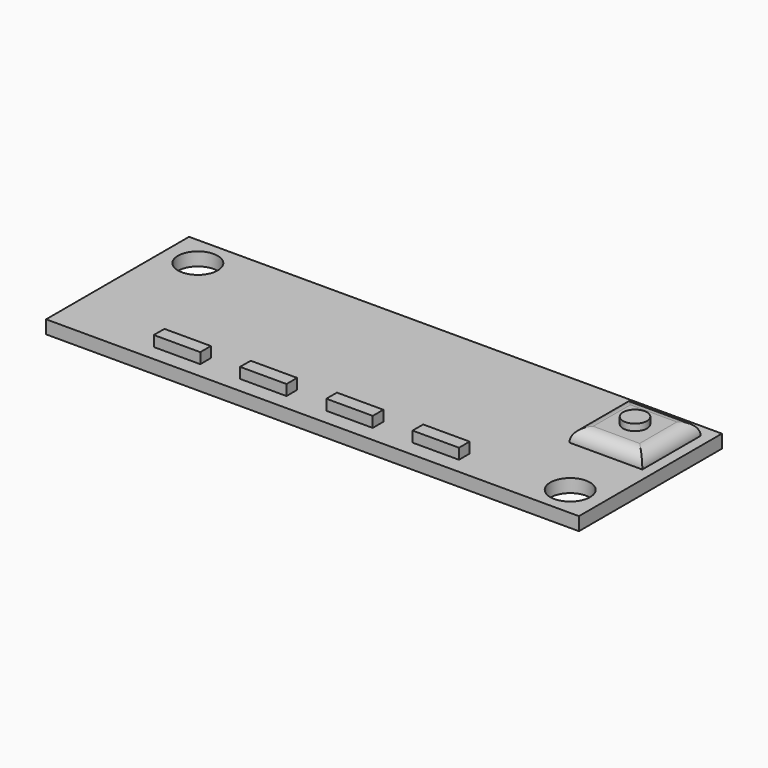
from build123d import *

# Parameters (mm, degrees)
F0_W     = 40.16
F0_H     = 13.47
F0_W_2   = 3.5
F0_H_2   = 1
F0_R     = 1.5
F0_W_3   = 5.5
F0_H_3   = 5.5
F1_DEPTH = 1
F2_DEPTH = 1.8
F3_DEPTH = 2
F4_R     = 0.99999
F5_R     = 0.9
F6_DEPTH = 0.5
F7_W     = 3
F7_H     = 8.5
F8_DEPTH = 1.2


# Not quite as in the source:
# - a fillet or chamfer is up to 0.001 mm smaller than in the source, because OpenCascade refuses the exact size


with BuildPart() as f1:
    # F0 (on Top) → F1 (new body)
    with BuildSketch(Plane.XY):
        with Locations((1.9053274065, 3.3154582972)):
            Rectangle(F0_W, F0_H)
        with Locations((-9.2646725935, -1.7195417028)):
            Rectangle(F0_W_2, F0_H_2, mode=Mode.SUBTRACT)
        with Locations((-2.7646725935, -1.7195417028)):
            Rectangle(F0_W_2, F0_H_2, mode=Mode.SUBTRACT)
        with Locations((3.7353274065, -1.7195417028)):
            Rectangle(F0_W_2, F0_H_2, mode=Mode.SUBTRACT)
        with Locations((10.2353274065, -1.7195417028)):
            Rectangle(F0_W_2, F0_H_2, mode=Mode.SUBTRACT)
        with Locations((19.4853274065, -1.1195417028)):
            Circle(F0_R, mode=Mode.SUBTRACT)
        with Locations((-15.6746725935, 7.7504582972)):
            Circle(F0_R, mode=Mode.SUBTRACT)
        with Locations((18.4353274065, 6.3004582972)):
            Rectangle(F0_W_3, F0_H_3, mode=Mode.SUBTRACT)
        with Locations((-9.2646725935, -1.7195417028)):
            Rectangle(F0_W_2, F0_H_2)
        with Locations((-2.7646725935, -1.7195417028)):
            Rectangle(F0_W_2, F0_H_2)
        with Locations((3.7353274065, -1.7195417028)):
            Rectangle(F0_W_2, F0_H_2)
        with Locations((10.2353274065, -1.7195417028)):
            Rectangle(F0_W_2, F0_H_2)
        with Locations((18.4353274065, 6.3004582972)):
            Rectangle(F0_W_3, F0_H_3)
    extrude(amount=F1_DEPTH)

    # F0 (on Top) → F2 (join)
    with BuildSketch(Plane.XY):
        with Locations((-9.2646725935, -1.7195417028)):
            Rectangle(F0_W_2, F0_H_2)
        with Locations((-2.7646725935, -1.7195417028)):
            Rectangle(F0_W_2, F0_H_2)
        with Locations((3.7353274065, -1.7195417028)):
            Rectangle(F0_W_2, F0_H_2)
        with Locations((10.2353274065, -1.7195417028)):
            Rectangle(F0_W_2, F0_H_2)
    extrude(amount=F2_DEPTH)

    # F0 (on Top) → F3 (join)
    with BuildSketch(Plane.XY):
        with Locations((18.4353274065, 6.3004582972)):
            Rectangle(F0_W_3, F0_H_3)
    extrude(amount=F3_DEPTH)

    # F4 (radius 1 in the source; OpenCascade refuses exactly that, so slightly less here)
    f4_edges = [f1.edges().sort_by_distance(p)[0] for p in [
        (21.185327, 6.300458, 2),
        (15.685327, 6.300458, 2),
        (18.435327, 3.550458, 2),
        (18.435327, 9.050458, 2),
    ]]
    fillet(f4_edges, radius=F4_R)

    # F5 (on face) → F6 (join)
    with BuildSketch(Plane.XY.offset(2)):
        with Locations((18.4353274065, 6.3004582972)):
            Circle(F5_R)
    extrude(amount=F6_DEPTH)

    # F7 (on face) → F8 (join)
    with BuildSketch(Plane(origin=(0, 0, 0), x_dir=(1, 0, 0), z_dir=(0, 0, -1))):
        with Locations((-1.5146725935, -4.8004582972)):
            Rectangle(F7_W, F7_H)
    extrude(amount=F8_DEPTH)


solid = f1.part
